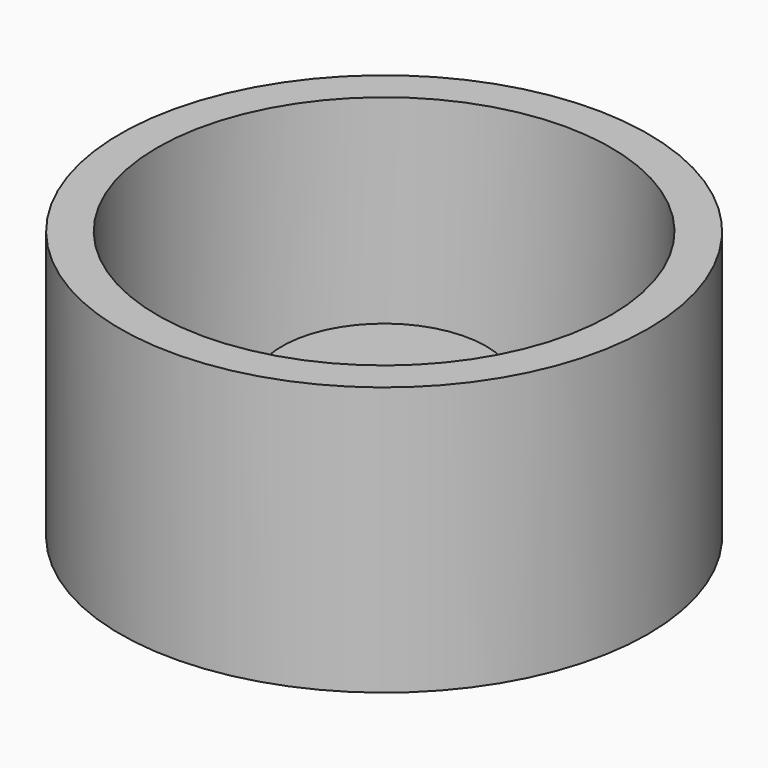
from build123d import *

# Parameters (mm, degrees)
F0_R     = 49.900321063
F0_R_2   = 42.8719097742
F1_DEPTH = 50.8
F2_R     = 19.3101591149
F3_DEPTH = 25.4


# Not quite as in the source:
# - a feature names something its author has since deleted; it is built from what else it names


with BuildPart() as f1:
    # F0 (on Top) → F1 (new body)
    with BuildSketch(Plane.XY):
        Circle(F0_R)
        Circle(F0_R_2, mode=Mode.SUBTRACT)
    extrude(amount=F1_DEPTH)


with BuildPart() as f3:
    # F2 (on Top) → F3 (new body)
    with BuildSketch(Plane.XY):
        Circle(F2_R)
    extrude(amount=F3_DEPTH)


solid = Compound([f1.part, f3.part])
